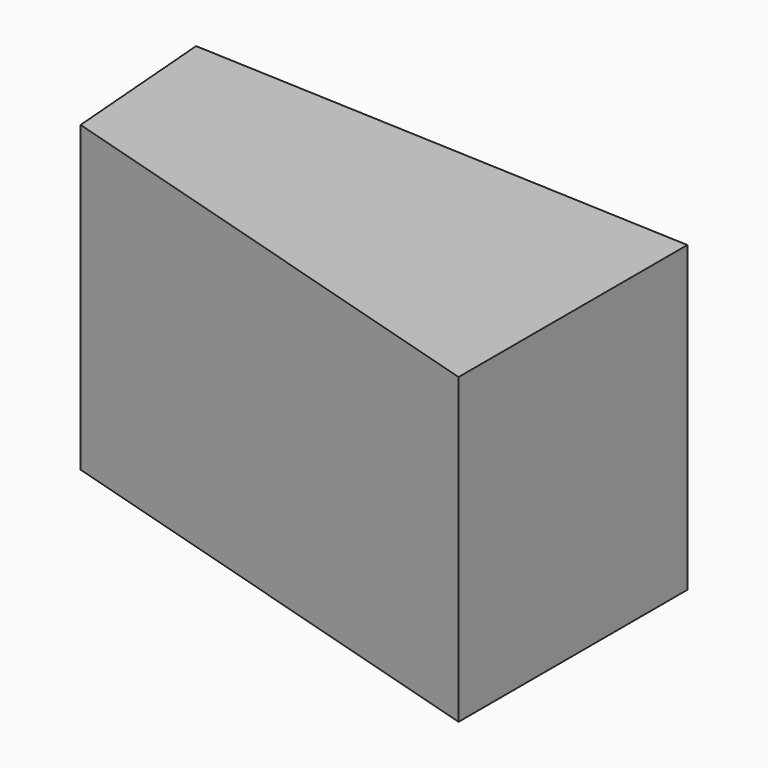
from build123d import *

# Parameters (mm, degrees)
F1_DEPTH = 52.53632


# Not quite as in the source:
# - a feature names something its author has since deleted; it is built from what else it names


with BuildPart() as f1:
    # F0 (on Top) → F1 (new body, symmetric)
    with BuildSketch(Plane.XY):
        Polygon((-117.4078658223, 55.4891340435), (-112.9749193788, 0), (58.9966401458, -51.4805689454), (58.9966401458, 47.5227497518), align=None)
    extrude(amount=F1_DEPTH, both=True)


solid = f1.part
